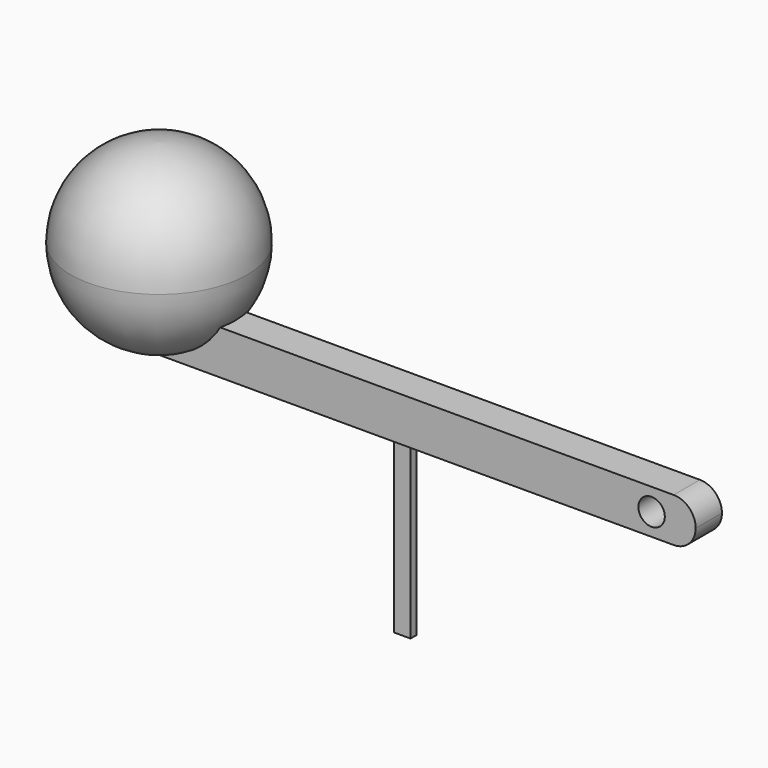
from build123d import *

# Parameters (mm, degrees)
F0_R     = 10
F1_DEPTH = 20
F2_R     = 9.99999
F3_W     = 62.343750149
F3_H     = 3.7187503185
F4_DEPTH = 5
F5_R     = 1.5004268613
F6_DEPTH = 25
F7_R     = 2.49999
F8_W     = 1.8586194401
F8_H     = 0.8482741494
F9_DEPTH = 20


# Not quite as in the source:
# - a fillet or chamfer is up to 0.001 mm smaller than in the source, because OpenCascade refuses the exact size


with BuildPart() as f1:
    # F0 (on Top) → F1 (new body)
    with BuildSketch(Plane.XY):
        Circle(F0_R)
    extrude(amount=F1_DEPTH)

    # F2 (radius 10 in the source; OpenCascade refuses exactly that, so slightly less here)
    f2_edges = [f1.edges().sort_by_distance(p)[0] for p in [
        (-10, 0, 20),
        (-10, 0, 0),
    ]]
    fillet(f2_edges, radius=F2_R)


with BuildPart() as f4:
    # F3 (on Top) → F4 (new body)
    with BuildSketch(Plane.XY):
        with Locations((31.1718750745, 0)):
            Rectangle(F3_W, F3_H)
    extrude(amount=F4_DEPTH)

    # F5 (on face) → F6 (cut)
    with BuildSketch(Plane.XZ.offset(1.8593751593)):
        with Locations((57.343750149, 2.5)):
            Circle(F5_R)
    extrude(amount=-F6_DEPTH, mode=Mode.SUBTRACT)

    # F7 (radius 2.5 in the source; OpenCascade refuses exactly that, so slightly less here)
    f7_edges = [f4.edges().sort_by_distance(p)[0] for p in [
        (62.34375, 0, 0),
        (62.34375, 0, 5),
    ]]
    fillet(f7_edges, radius=F7_R)

    # F8 (on face) → F9 (join)
    with BuildSketch(Plane(origin=(0, 0, 0), x_dir=(1, 0, 0), z_dir=(0, 0, -1))):
        with Locations((27.92930972, 0)):
            Rectangle(F8_W, F8_H)
    extrude(amount=F9_DEPTH)


solid = Compound([f1.part, f4.part])
